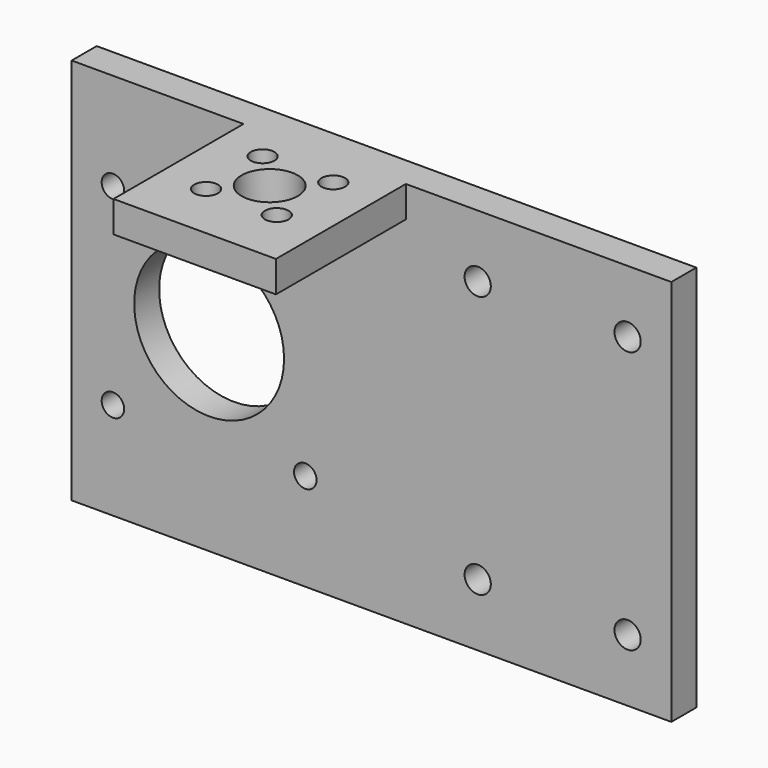
from build123d import *

# Parameters (mm, degrees)
F0_W     = 96
F0_H     = 62
F0_R     = 1.8
F0_R_2   = 2.1
F0_R_3   = 12
F1_DEPTH = 5
F2_W     = 26
F2_H     = 5
F3_DEPTH = 26
F4_R     = 4.5
F4_R_2   = 1.8935291465
F5_DEPTH = 25


# Not quite as in the source:
# - a feature names something its author has since deleted; it is built from what else it names


with BuildPart() as f1:
    # F0 (on Front) → F1 (new body)
    with BuildSketch(Plane.XZ):
        with Locations((0, 31)):
            Rectangle(F0_W, F0_H)
        with Locations((-41.4, 15.6001571745)):
            Circle(F0_R, mode=Mode.SUBTRACT)
        with Locations((-10.6, 15.6001571745)):
            Circle(F0_R, mode=Mode.SUBTRACT)
        with Locations((17, 10)):
            Circle(F0_R_2, mode=Mode.SUBTRACT)
        with Locations((41, 10)):
            Circle(F0_R_2, mode=Mode.SUBTRACT)
        with Locations((-26, 31)):
            Circle(F0_R_3, mode=Mode.SUBTRACT)
        with Locations((-41.4, 46.4001571745)):
            Circle(F0_R, mode=Mode.SUBTRACT)
        with Locations((-10.6, 46.4001571745)):
            Circle(F0_R, mode=Mode.SUBTRACT)
        with Locations((17, 52)):
            Circle(F0_R_2, mode=Mode.SUBTRACT)
        with Locations((41, 52)):
            Circle(F0_R_2, mode=Mode.SUBTRACT)
    extrude(amount=F1_DEPTH)

    # F2 (on face) → F3 (join)
    with BuildSketch(Plane.XZ.offset(5)):
        with Locations((-7.5, 59.5)):
            Rectangle(F2_W, F2_H)
    extrude(amount=F3_DEPTH)

    # F4 (on face) → F5 (cut)
    with BuildSketch(Plane.XY.offset(62)):
        with Locations((-7.5, -16)):
            Circle(F4_R)
        with Locations((-13.1568542495, -10.3431457505)):
            Circle(F4_R_2)
        with Locations((-1.8431457505, -10.3431457505)):
            Circle(F4_R_2)
        with Locations((-1.8431457505, -21.6568542495)):
            Circle(F4_R_2)
        with Locations((-13.1568542495, -21.6568542495)):
            Circle(F4_R_2)
    extrude(amount=-F5_DEPTH, mode=Mode.SUBTRACT)


solid = f1.part
